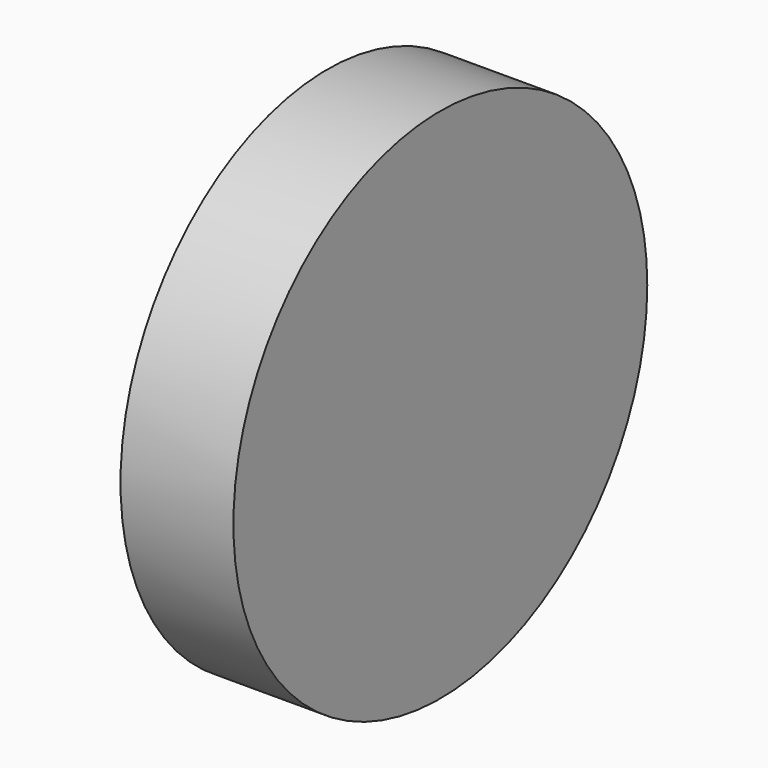
from build123d import *

# Parameters (mm, degrees)
F0_R     = 58.1989244335
F2_DEPTH = 25.4


# Not quite as in the source:
# - the program builds the solid bodies; features that only make, move or delete a surface that nothing else refers to are left out


with BuildPart() as f2:
    # F0 (on Right) → F2 (new body)
    with BuildSketch(Plane.YZ):
        with Locations((0, -35.8079969883)):
            Circle(F0_R)
    extrude(amount=F2_DEPTH)


solid = f2.part
